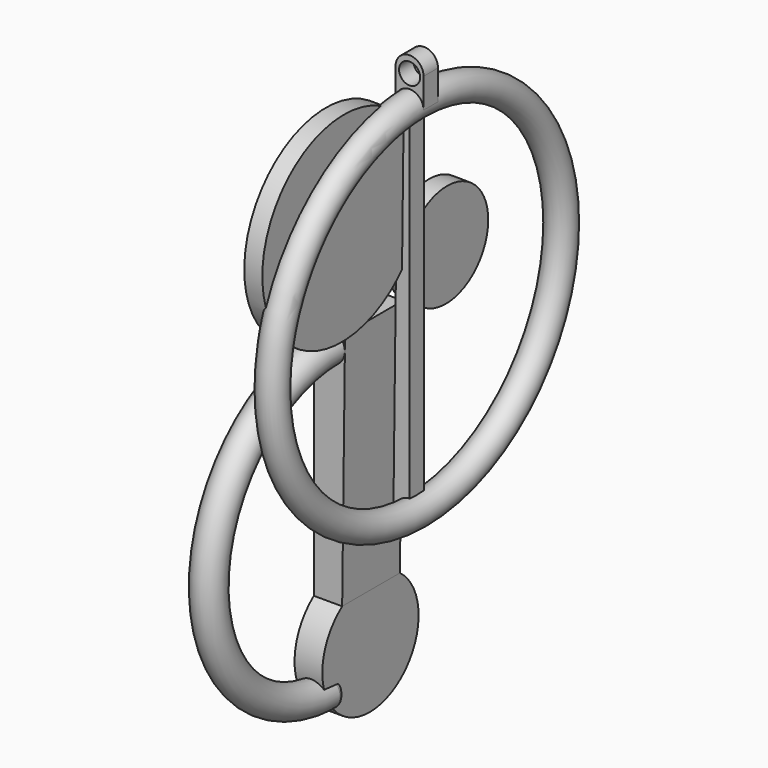
from build123d import *

# Parameters (mm, degrees)
F0_R          = 2.3255601838
F3_DEPTH      = 12
F4_R          = 10
F5_REACH      = 38.1287390872
F6_R          = 2.5805347307
F7_ANGLE      = 180
F9_DEPTH      = 2
F9_DEPTH_BACK = 1
F10_W         = 3
F10_H         = 58.6224048207
F11_REACH     = 66.2180248443
F13_R         = 1
F12_R         = 1.75
F14_DEPTH     = 1.5


with BuildPart() as f1:
    # F0 (on Front) → F1 (revolve)
    with BuildSketch(Plane.XZ):
        with Locations((0, 30)):
            Circle(F0_R)
    revolve(axis=Axis((-0.4632313671, 0, 0), (1, 0, 0)))

    # F8 (on face) → F9 (join, two sides)
    with BuildSketch(Plane(origin=(-2.3252226581, 0, 0.0280146809), x_dir=(0, 1, 0), z_dir=(0.9999274287, 0, -0.0120472969))) as f9_sk:
        with BuildLine():
            ThreePointArc((2.0805130523, 11.9105497142), (2.5910354273, 14.2497875874), (2.7623795628, 16.6379475716))
            ThreePointArc((2.7623795628, 16.6379475716), (-29.7588639596, 22.1545713112), (-0.8760942598, 6.2218994639))
            ThreePointArc((-0.8760942598, 6.2218994639), (0.0568757564, 9.3496551669), (2.0805130523, 11.9105497142))
        make_face()
        with BuildLine():
            ThreePointArc((2.0805130523, 11.9105497142), (0.8772757251, 8.9232621844), (-0.8760942598, 6.2218994639))
            ThreePointArc((-0.8760942598, 6.2218994639), (7.312045103, -3.303341458), (16.4141692485, 5.3527071141))
            ThreePointArc((16.4141692485, 5.3527071141), (11.3529879248, 13.2339982443), (2.0805130523, 11.9105497142))
        make_face()
        with BuildLine():
            ThreePointArc((2.0805130523, 11.9105497142), (0.0568757564, 9.3496551669), (-0.8760942598, 6.2218994639))
            ThreePointArc((-0.8760942598, 6.2218994639), (0.8772757251, 8.9232621844), (2.0805130523, 11.9105497142))
        make_face()
    extrude(amount=-F9_DEPTH)
    extrude(f9_sk.sketch, amount=F9_DEPTH_BACK)


with BuildPart() as f3:
    # F2 (on Front) → F3 (new body)
    with BuildSketch(Plane.XZ):
        Polygon((-2.8074870352, -40), (-2.3255601838, 0), (-7.5179076559, 0), (-7.5179076559, -40), align=None)
    extrude(amount=F3_DEPTH)

    f5_end = Plane(origin=(-2.5665236095, -6, -20), x_dir=(0.0120472969, 0, 0.9999274287), z_dir=(0.9999274287, 0, -0.0120472969))
    # F4 (on face) → F5 (join, up to a plane its end follows)
    with BuildSketch(Plane(origin=(-7.5179076559, 0, 0), x_dir=(0, -1, 0), z_dir=(-1, 0, 0))):
        with Locations((6, -48)):
            Circle(F4_R)
    f5_long = extrude(amount=-F5_REACH, mode=Mode.PRIVATE)
    add(split(f5_long, bisect_by=f5_end, keep=Keep.BOTTOM, mode=Mode.PRIVATE))


with BuildPart() as f7:
    # F6 (on face) → F7 (revolve)
    with BuildSketch(Plane.XZ.offset(12)):
        with Locations((-4.9373729253, -2.5805347307)):
            Circle(F6_R)
    revolve(axis=Axis((0.6807111204, -12, -27.6477448642), (1, 0, 0)), revolution_arc=F7_ANGLE)

    # F13
    f13_edges = [f7.edges().sort_by_distance(p)[0] for p in [
        (-7.517908, -12, -52.714955),
    ]]
    fillet(f13_edges, radius=F13_R)


with BuildPart() as f11:
    f11_end = Plane(origin=(-2.697918947, -6, -30.9058324611), x_dir=(0.0120472969, 0, 0.9999274287), z_dir=(0.9999274287, 0, -0.0120472969))
    # F10 (on Right) → F11 (new body, up to a plane its end follows)
    with BuildSketch(Plane.YZ):
        with Locations((0, 0.1569753513)):
            Rectangle(F10_W, F10_H)
    f11_long = extrude(amount=-F11_REACH, mode=Mode.PRIVATE)
    add(split(f11_long, bisect_by=f11_end, keep=Keep.TOP, mode=Mode.PRIVATE))


with BuildPart() as f14:
    # F12 (on Front) → F14 (new body, symmetric)
    with BuildSketch(Plane.XZ):
        with BuildLine():
            ThreePointArc((-2.3255601838, 30), (0, 32.3255601838), (2.3255601838, 30))
            Line((2.3255601838, 30), (2.3255601838, 34.9638313055))
            ThreePointArc((2.3255601838, 34.9638313055), (0, 37.2893914893), (-2.3255601838, 34.9638313055))
            Line((-2.3255601838, 34.9638313055), (-2.3255601838, 30))
        make_face()
        with Locations((0, 34.6128940582)):
            Circle(F12_R, mode=Mode.SUBTRACT)
    extrude(amount=F14_DEPTH, both=True)


solid = Compound([f1.part, f3.part, f7.part, f11.part, f14.part])
